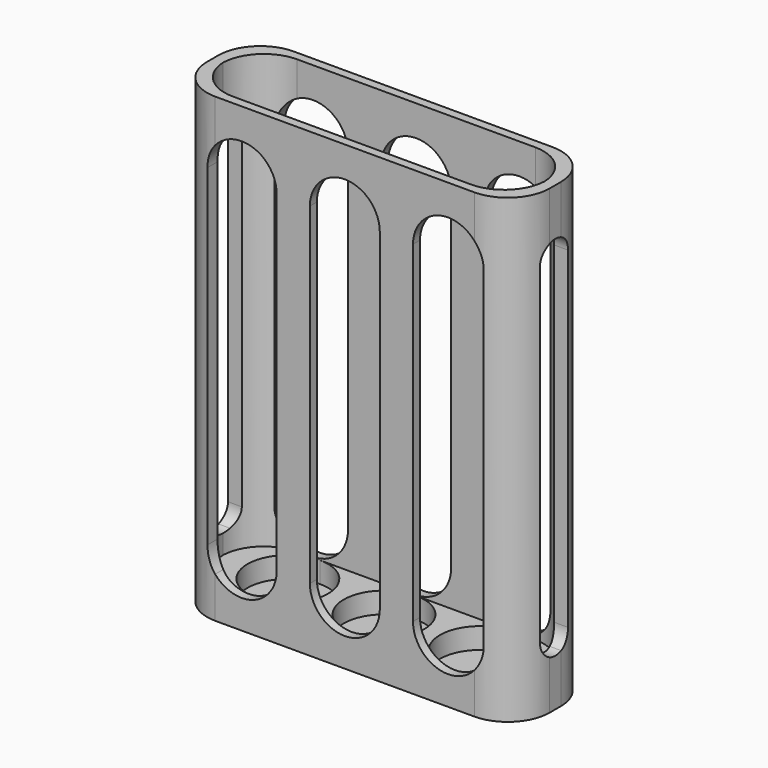
from build123d import *

# Parameters (mm, degrees)
F0_W         = 98
F0_H         = 28
F1_DEPTH     = 2
F2_DEPTH     = 130
F3_T4_DEPTH  = 160.0024142302
F3_T9_DEPTH  = 160.0024142302
F3_T14_DEPTH = 160.0024142302
F3_T19_DEPTH = 160.0024142302
F3_T21_DEPTH = 192.0048284605
F4_W         = 17.5970186629
F4_H         = 95
F4_W_2       = 2.4029813371
F4_W_3       = 20
F5_DEPTH     = 50
F6_W         = 2.9029813371
F6_H         = 95
F6_W_2       = 4.1940373259
F7_DEPTH     = 100
F9_DEPTH     = 6


# Not quite as in the source:
# - a fillet or chamfer that OpenCascade refuses, or shapes differently, is made with other operations: its cross-section is extruded or revolved along the edge and cut away or added


with BuildPart() as f1:
    # F0 (on Top) → F1 (new body)
    with BuildSketch(Plane.XY):
        Rectangle(F0_W, F0_H)
        Polygon((-46, 11.5), (-34.5, 11.5), (-11.5, 11.5), (11.4999999714, 11.5), (34.5, 11.5), (46, 11.5), (46, 0), (46, -11.5), (34.5, -11.5), (11.4999998877, -11.5), (-11.5, -11.5), (-34.5, -11.5), (-46, -11.5), (-46, 0), align=None, mode=Mode.SUBTRACT)
        with BuildLine():
            Line((-34.5, 0), (-34.5, 11.5))
            ThreePointArc((-34.5, 11.5), (-42.6317279836, 8.1317279836), (-46, 0))
            Line((-46, 0), (-34.5, 0))
        make_face()
        with BuildLine():
            ThreePointArc((-46, 0), (-42.6317279836, -8.1317279836), (-34.5, -11.5))
            Line((-34.5, -11.5), (-34.5, 0))
            Line((-34.5, 0), (-46, 0))
        make_face()
        with BuildLine():
            ThreePointArc((-34.5, -11.5), (-26.3682720164, -8.1317279836), (-23, 0))
            ThreePointArc((-23, 0), (-26.3682720164, 8.1317279836), (-34.5, 11.5))
            Line((-34.5, 11.5), (-34.5, 0))
            Line((-34.5, 0), (-34.5, -11.5))
        make_face()
        with BuildLine():
            ThreePointArc((-11.5, -11.5), (-19.6317279836, -8.1317279836), (-23, 0))
            ThreePointArc((-23, 0), (-26.3682720164, -8.1317279836), (-34.5, -11.5))
            Line((-34.5, -11.5), (-11.5, -11.5))
        make_face()
        with BuildLine():
            ThreePointArc((-11.5, 11.5), (-19.6317279836, 8.1317279836), (-23, 0))
            ThreePointArc((-23, 0), (-19.6317279836, -8.1317279836), (-11.5, -11.5))
            ThreePointArc((-11.5, -11.5), (-3.3682720164, -8.1317279836), (0, 0))
            ThreePointArc((0, 0), (-3.3682720164, 8.1317279836), (-11.5, 11.5))
        make_face()
        with BuildLine():
            ThreePointArc((-34.5, 11.5), (-26.3682720164, 8.1317279836), (-23, 0))
            ThreePointArc((-23, 0), (-19.6317279836, 8.1317279836), (-11.5, 11.5))
            Line((-11.5, 11.5), (-34.5, 11.5))
        make_face()
        with BuildLine():
            ThreePointArc((0, 0), (-3.3682720164, -8.1317279836), (-11.5, -11.5))
            Line((-11.5, -11.5), (11.4999998877, -11.5))
            ThreePointArc((11.4999998877, -11.5), (3.3682719767, -8.131727944), (0, 0))
        make_face()
        with BuildLine():
            Line((11.4999999714, 11.5), (-11.5, 11.5))
            ThreePointArc((-11.5, 11.5), (-3.3682720164, 8.1317279836), (0, 0))
            ThreePointArc((0, 0), (3.3682720062, 8.1317279735), (11.4999999714, 11.5))
        make_face()
        with BuildLine():
            ThreePointArc((11.4999999714, 11.5), (3.3682720062, 8.1317279735), (0, 0))
            ThreePointArc((0, 0), (3.3682719767, -8.131727944), (11.4999998877, -11.5))
            ThreePointArc((11.4999998877, -11.5), (19.631727944, -8.1317280233), (23, 0))
            ThreePointArc((23, 0), (19.6317279735, 8.1317279938), (11.4999999714, 11.5))
        make_face()
        with BuildLine():
            ThreePointArc((34.5, 11.5), (26.3682720164, 8.1317279836), (23, 0))
            ThreePointArc((23, 0), (26.3682720164, -8.1317279836), (34.5, -11.5))
            Line((34.5, -11.5), (34.5, 0))
            Line((34.5, 0), (34.5, 11.5))
        make_face()
        with BuildLine():
            ThreePointArc((46, 0), (42.6317279836, 8.1317279836), (34.5, 11.5))
            Line((34.5, 11.5), (34.5, 0))
            Line((34.5, 0), (46, 0))
        make_face()
        with BuildLine():
            Line((34.5, 0), (34.5, -11.5))
            ThreePointArc((34.5, -11.5), (42.6317279836, -8.1317279836), (46, 0))
            Line((46, 0), (34.5, 0))
        make_face()
        with BuildLine():
            ThreePointArc((23, 0), (19.631727944, -8.1317280233), (11.4999998877, -11.5))
            Line((11.4999998877, -11.5), (34.5, -11.5))
            ThreePointArc((34.5, -11.5), (26.3682720164, -8.1317279836), (23, 0))
        make_face()
        with BuildLine():
            Line((34.5, 11.5), (11.4999999714, 11.5))
            ThreePointArc((11.4999999714, 11.5), (19.6317279735, 8.1317279938), (23, 0))
            ThreePointArc((23, 0), (26.3682720164, 8.1317279836), (34.5, 11.5))
        make_face()
        with BuildLine():
            Line((-46, -11.5), (-34.5, -11.5))
            ThreePointArc((-34.5, -11.5), (-42.6317279836, -8.1317279836), (-46, 0))
            Line((-46, 0), (-46, -11.5))
        make_face()
        with BuildLine():
            ThreePointArc((-46, 0), (-42.6317279836, 8.1317279836), (-34.5, 11.5))
            Line((-34.5, 11.5), (-46, 11.5))
            Line((-46, 11.5), (-46, 0))
        make_face()
        with BuildLine():
            Line((46, 11.5), (34.5, 11.5))
            ThreePointArc((34.5, 11.5), (42.6317279836, 8.1317279836), (46, 0))
            Line((46, 0), (46, 11.5))
        make_face()
        with BuildLine():
            ThreePointArc((46, 0), (42.6317279836, -8.1317279836), (34.5, -11.5))
            Line((34.5, -11.5), (46, -11.5))
            Line((46, -11.5), (46, 0))
        make_face()
    extrude(amount=-F1_DEPTH)

    # F0 (on Top) → F2 (join)
    with BuildSketch(Plane.XY):
        Rectangle(F0_W, F0_H)
        Polygon((-46, 11.5), (-34.5, 11.5), (-11.5, 11.5), (11.4999999714, 11.5), (34.5, 11.5), (46, 11.5), (46, 0), (46, -11.5), (34.5, -11.5), (11.4999998877, -11.5), (-11.5, -11.5), (-34.5, -11.5), (-46, -11.5), (-46, 0), align=None, mode=Mode.SUBTRACT)
    extrude(amount=F2_DEPTH)

    # F3: fillet of radius 12 on 8 edges, made by hand


with BuildPart() as f3_tool2:
    # F3_s3 → F3_t4 (new body)
    with BuildSketch(Plane.XY.offset(-30.0024142302)):
        with BuildLine():
            ThreePointArc((46.0004, -0.5009656854), (42.4852813742, 7.9852813742), (33.9990343146, 11.5004))
            Line((33.9990343146, 11.5004), (33.9990343146, 12.7005365685))
            ThreePointArc((33.9990343146, 12.7005365685), (39.9995171573, 12.7001365685), (46, 12.7001365685))
            Line((46, 12.7001365685), (47.2001365685, 11.5))
            ThreePointArc((47.2001365685, 11.5), (47.2001365685, 5.4995171573), (47.2005365685, -0.5009656854))
            Line((47.2005365685, -0.5009656854), (46.0004, -0.5009656854))
        make_face()
    extrude(amount=F3_T4_DEPTH)

    split(bisect_by=Plane.XY.offset(-2), keep=Keep.TOP)


with BuildPart() as f1_1:
    add(f1.part)

    # F3_t1: union F3_tool2
    add(f3_tool2.part)


with BuildPart() as f3_tool7:
    # F3_s8 → F3_t9 (new body)
    with BuildSketch(Plane.XY.offset(-30.0024142302)):
        with BuildLine():
            ThreePointArc((33.9990343146, -11.5004), (42.4852813742, -7.9852813742), (46.0004, 0.5009656854))
            Line((46.0004, 0.5009656854), (47.2005365685, 0.5009656854))
            ThreePointArc((47.2005365685, 0.5009656854), (47.2001365685, -5.4995171573), (47.2001365685, -11.5))
            Line((47.2001365685, -11.5), (46, -12.7001365685))
            ThreePointArc((46, -12.7001365685), (39.9995171573, -12.7001365685), (33.9990343146, -12.7005365685))
            Line((33.9990343146, -12.7005365685), (33.9990343146, -11.5004))
        make_face()
    extrude(amount=F3_T9_DEPTH)

    split(bisect_by=Plane.XY.offset(-2), keep=Keep.TOP)


with BuildPart() as f1_2:
    add(f1_1.part)

    # F3_t6: union F3_tool7
    add(f3_tool7.part)


with BuildPart() as f3_tool12:
    # F3_s13 → F3_t14 (new body)
    with BuildSketch(Plane.XY.offset(-30.0024142302)):
        with BuildLine():
            ThreePointArc((-46.0004, -0.5009656854), (-42.4852813742, 7.9852813742), (-33.9990343146, 11.5004))
            Line((-33.9990343146, 11.5004), (-33.9990343146, 12.7005365685))
            ThreePointArc((-33.9990343146, 12.7005365685), (-39.9995171573, 12.7001365685), (-46, 12.7001365685))
            Line((-46, 12.7001365685), (-47.2001365685, 11.5))
            ThreePointArc((-47.2001365685, 11.5), (-47.2001365685, 5.4995171573), (-47.2005365685, -0.5009656854))
            Line((-47.2005365685, -0.5009656854), (-46.0004, -0.5009656854))
        make_face()
    extrude(amount=F3_T14_DEPTH)

    split(bisect_by=Plane.XY.offset(-2), keep=Keep.TOP)


with BuildPart() as f1_3:
    add(f1_2.part)

    # F3_t11: union F3_tool12
    add(f3_tool12.part)


with BuildPart() as f3_tool17:
    # F3_s18 → F3_t19 (new body)
    with BuildSketch(Plane.XY.offset(-30.0024142302)):
        with BuildLine():
            ThreePointArc((-46.0004, 0.5009656854), (-42.4852813742, -7.9852813742), (-33.9990343146, -11.5004))
            Line((-33.9990343146, -11.5004), (-33.9990343146, -12.7005365685))
            ThreePointArc((-33.9990343146, -12.7005365685), (-39.9995171573, -12.7001365685), (-46, -12.7001365685))
            Line((-46, -12.7001365685), (-47.2001365685, -11.5))
            ThreePointArc((-47.2001365685, -11.5), (-47.2001365685, -5.4995171573), (-47.2005365685, 0.5009656854))
            Line((-47.2005365685, 0.5009656854), (-46.0004, 0.5009656854))
        make_face()
    extrude(amount=F3_T19_DEPTH)

    split(bisect_by=Plane.XY.offset(-2), keep=Keep.TOP)


with BuildPart() as f1_4:
    add(f1_3.part)

    # F3_t16: union F3_tool17
    add(f3_tool17.part)

    # F3_s22 → F3_t21 (cut)
    with BuildSketch(Plane.XY.offset(-32.0024142302)):
        with BuildLine():
            ThreePointArc((-36.9990343146, 14.0004), (-45.4852813742, 10.4852813742), (-49.0004, 1.9990343146))
            Line((-49.0004, 1.9990343146), (-50.2005365685, 1.9990343146))
            ThreePointArc((-50.2005365685, 1.9990343146), (-50.2001365685, 7.9995171573), (-50.2001365685, 14))
            Line((-50.2001365685, 14), (-49, 15.2001365685))
            ThreePointArc((-49, 15.2001365685), (-42.9995171573, 15.2001365685), (-36.9990343146, 15.2005365685))
            Line((-36.9990343146, 15.2005365685), (-36.9990343146, 14.0004))
        make_face()
        with BuildLine():
            ThreePointArc((-36.9990343146, -14.0004), (-45.4852813742, -10.4852813742), (-49.0004, -1.9990343146))
            Line((-49.0004, -1.9990343146), (-50.2005365685, -1.9990343146))
            ThreePointArc((-50.2005365685, -1.9990343146), (-50.2001365685, -7.9995171573), (-50.2001365685, -14))
            Line((-50.2001365685, -14), (-49, -15.2001365685))
            ThreePointArc((-49, -15.2001365685), (-42.9995171573, -15.2001365685), (-36.9990343146, -15.2005365685))
            Line((-36.9990343146, -15.2005365685), (-36.9990343146, -14.0004))
        make_face()
        with BuildLine():
            ThreePointArc((49.0004, -1.9990343146), (45.4852813742, -10.4852813742), (36.9990343146, -14.0004))
            Line((36.9990343146, -14.0004), (36.9990343146, -15.2005365685))
            ThreePointArc((36.9990343146, -15.2005365685), (42.9995171573, -15.2001365685), (49, -15.2001365685))
            Line((49, -15.2001365685), (50.2001365685, -14))
            ThreePointArc((50.2001365685, -14), (50.2001365685, -7.9995171573), (50.2005365685, -1.9990343146))
            Line((50.2005365685, -1.9990343146), (49.0004, -1.9990343146))
        make_face()
        with BuildLine():
            ThreePointArc((49.0004, 1.9990343146), (45.4852813742, 10.4852813742), (36.9990343146, 14.0004))
            Line((36.9990343146, 14.0004), (36.9990343146, 15.2005365685))
            ThreePointArc((36.9990343146, 15.2005365685), (42.9995171573, 15.2001365685), (49, 15.2001365685))
            Line((49, 15.2001365685), (50.2001365685, 14))
            ThreePointArc((50.2001365685, 14), (50.2001365685, 7.9995171573), (50.2005365685, 1.9990343146))
            Line((50.2005365685, 1.9990343146), (49.0004, 1.9990343146))
        make_face()
    extrude(amount=F3_T21_DEPTH, mode=Mode.SUBTRACT)

    # F4 (on face) → F5 (cut)
    with BuildSketch(Plane.XZ.offset(14)):
        with Locations((-28.2985093315, 63.7274757028)):
            Rectangle(F4_W, F4_H)
        with Locations((-38.2985093315, 63.7274757028)):
            Rectangle(F4_W_2, F4_H)
        with BuildLine():
            Line((-37.0970186629, 111.2274757028), (-19.5, 111.2274757028))
            ThreePointArc((-19.5, 111.2274757028), (-26.0337474579, 120.6075126598), (-37.0970186629, 117.7301910921))
            Line((-37.0970186629, 117.7301910921), (-37.0970186629, 111.2274757028))
        make_face()
        with BuildLine():
            Line((-39.5, 111.2274757028), (-37.0970186629, 111.2274757028))
            Line((-37.0970186629, 111.2274757028), (-37.0970186629, 117.7301910921))
            ThreePointArc((-37.0970186629, 117.7301910921), (-38.880036957, 114.6937282448), (-39.5, 111.2274757028))
        make_face()
        with BuildLine():
            ThreePointArc((10, 111.2274757028), (0, 121.2274757028), (-10, 111.2274757028))
            Line((-10, 111.2274757028), (10, 111.2274757028))
        make_face()
        with Locations((0, 63.7274757028)):
            Rectangle(F4_W_3, F4_H)
        with BuildLine():
            ThreePointArc((-37.0970186629, 9.7247603134), (-26.0337474579, 6.8474387458), (-19.5, 16.2274757028))
            Line((-19.5, 16.2274757028), (-37.0970186629, 16.2274757028))
            Line((-37.0970186629, 16.2274757028), (-37.0970186629, 9.7247603134))
        make_face()
        with BuildLine():
            Line((-37.0970186629, 9.7247603134), (-37.0970186629, 16.2274757028))
            Line((-37.0970186629, 16.2274757028), (-39.5, 16.2274757028))
            ThreePointArc((-39.5, 16.2274757028), (-38.880036957, 12.7612231607), (-37.0970186629, 9.7247603134))
        make_face()
        with BuildLine():
            Line((10, 16.2274757028), (-10, 16.2274757028))
            ThreePointArc((-10, 16.2274757028), (0, 6.2274757028), (10, 16.2274757028))
        make_face()
        with BuildLine():
            ThreePointArc((19.5, 16.2274757028), (26.0337474579, 6.8474387458), (37.0970186629, 9.7247603134))
            Line((37.0970186629, 9.7247603134), (37.0970186629, 16.2274757028))
            Line((37.0970186629, 16.2274757028), (19.5, 16.2274757028))
        make_face()
        with BuildLine():
            Line((37.0970186629, 16.2274757028), (37.0970186629, 9.7247603134))
            ThreePointArc((37.0970186629, 9.7247603134), (38.880036957, 12.7612231607), (39.5, 16.2274757028))
            Line((39.5, 16.2274757028), (37.0970186629, 16.2274757028))
        make_face()
        with Locations((38.2985093315, 63.7274757028)):
            Rectangle(F4_W_2, F4_H)
        with Locations((28.2985093315, 63.7274757028)):
            Rectangle(F4_W, F4_H)
        with BuildLine():
            Line((37.0970186629, 111.2274757028), (37.0970186629, 117.7301910921))
            ThreePointArc((37.0970186629, 117.7301910921), (26.0337474579, 120.6075126598), (19.5, 111.2274757028))
            Line((19.5, 111.2274757028), (37.0970186629, 111.2274757028))
        make_face()
        with BuildLine():
            ThreePointArc((39.5, 111.2274757028), (38.880036957, 114.6937282448), (37.0970186629, 117.7301910921))
            Line((37.0970186629, 117.7301910921), (37.0970186629, 111.2274757028))
            Line((37.0970186629, 111.2274757028), (39.5, 111.2274757028))
        make_face()
    extrude(amount=-F5_DEPTH, mode=Mode.SUBTRACT)

    # F6 (on face) → F7 (cut)
    with BuildSketch(Plane(origin=(-49, 0, 0), x_dir=(0, -1, 0), z_dir=(-1, 0, 0))):
        with BuildLine():
            Line((-5, 111.5), (-2.0970186629, 111.5))
            Line((-2.0970186629, 111.5), (-2.0970186629, 116.0389990887))
            ThreePointArc((-2.0970186629, 116.0389990887), (-4.2121902447, 114.193966099), (-5, 111.5))
        make_face()
        with BuildLine():
            Line((-2.0970186629, 111.5), (2.0970186629, 111.5))
            Line((2.0970186629, 111.5), (2.0970186629, 116.0389990887))
            ThreePointArc((2.0970186629, 116.0389990887), (0, 116.5), (-2.0970186629, 116.0389990887))
            Line((-2.0970186629, 116.0389990887), (-2.0970186629, 111.5))
        make_face()
        with Locations((3.5485093315, 64)):
            Rectangle(F6_W, F6_H)
        with Locations((0, 64)):
            Rectangle(F6_W_2, F6_H)
        with Locations((-3.5485093315, 64)):
            Rectangle(F6_W, F6_H)
        with BuildLine():
            Line((-2.0970186629, 11.9610009113), (-2.0970186629, 16.5))
            Line((-2.0970186629, 16.5), (-5, 16.5))
            ThreePointArc((-5, 16.5), (-4.2121902447, 13.806033901), (-2.0970186629, 11.9610009113))
        make_face()
        with BuildLine():
            Line((2.0970186629, 11.9610009113), (2.0970186629, 16.5))
            Line((2.0970186629, 16.5), (-2.0970186629, 16.5))
            Line((-2.0970186629, 16.5), (-2.0970186629, 11.9610009113))
            ThreePointArc((-2.0970186629, 11.9610009113), (0, 11.5), (2.0970186629, 11.9610009113))
        make_face()
        with BuildLine():
            ThreePointArc((2.0970186629, 11.9610009113), (4.2121902447, 13.806033901), (5, 16.5))
            Line((5, 16.5), (2.0970186629, 16.5))
            Line((2.0970186629, 16.5), (2.0970186629, 11.9610009113))
        make_face()
        with BuildLine():
            Line((2.0970186629, 111.5), (5, 111.5))
            ThreePointArc((5, 111.5), (4.2121902447, 114.193966099), (2.0970186629, 116.0389990887))
            Line((2.0970186629, 116.0389990887), (2.0970186629, 111.5))
        make_face()
    extrude(amount=-F7_DEPTH, mode=Mode.SUBTRACT)

    # F8 (on face) → F9 (join)
    with BuildSketch(Plane.XY):
        with BuildLine():
            ThreePointArc((-27.5, 11.5), (-19.3682720164, 8.1317279836), (-16, 0))
            ThreePointArc((-16, 0), (-19.3682720164, -8.1317279836), (-27.5, -11.5))
            Line((-27.5, -11.5), (-1.84e-08, -11.5))
            ThreePointArc((-1.84e-08, -11.5), (-11.5, 1.78e-08), (1.73e-08, 11.5))
            Line((1.73e-08, 11.5), (-27.5, 11.5))
        make_face()
        with BuildLine():
            ThreePointArc((-27.5, -11.5), (-39, 0), (-27.5, 11.5))
            Line((-27.5, 11.5), (-34.0970186629, 11.5))
            ThreePointArc((-34.0970186629, 11.5), (-42.341564727, 8.1266043452), (-45.9899396889, 0))
            ThreePointArc((-45.9899396889, 0), (-42.341564727, -8.1266043452), (-34.0970186629, -11.5))
            Line((-34.0970186629, -11.5), (-27.5, -11.5))
        make_face()
        with BuildLine():
            Line((27.5, 11.5), (1.73e-08, 11.5))
            ThreePointArc((1.73e-08, 11.5), (8.1317279898, 8.1317279775), (11.5, 0))
            ThreePointArc((11.5, 0), (8.1317279771, -8.1317279901), (-1.84e-08, -11.5))
            Line((-1.84e-08, -11.5), (27.5, -11.5))
            ThreePointArc((27.5, -11.5), (16, 0), (27.5, 11.5))
        make_face()
        with BuildLine():
            Line((34.0970186629, 11.5), (27.5, 11.5))
            ThreePointArc((27.5, 11.5), (35.6317279836, 8.1317279836), (39, 0))
            ThreePointArc((39, 0), (35.6317279836, -8.1317279836), (27.5, -11.5))
            Line((27.5, -11.5), (34.0970186629, -11.5))
            ThreePointArc((34.0970186629, -11.5), (42.341564727, -8.1266043452), (45.9899396889, 0))
            ThreePointArc((45.9899396889, 0), (42.341564727, 8.1266043452), (34.0970186629, 11.5))
        make_face()
    extrude(amount=F9_DEPTH)


solid = f1_4.part
